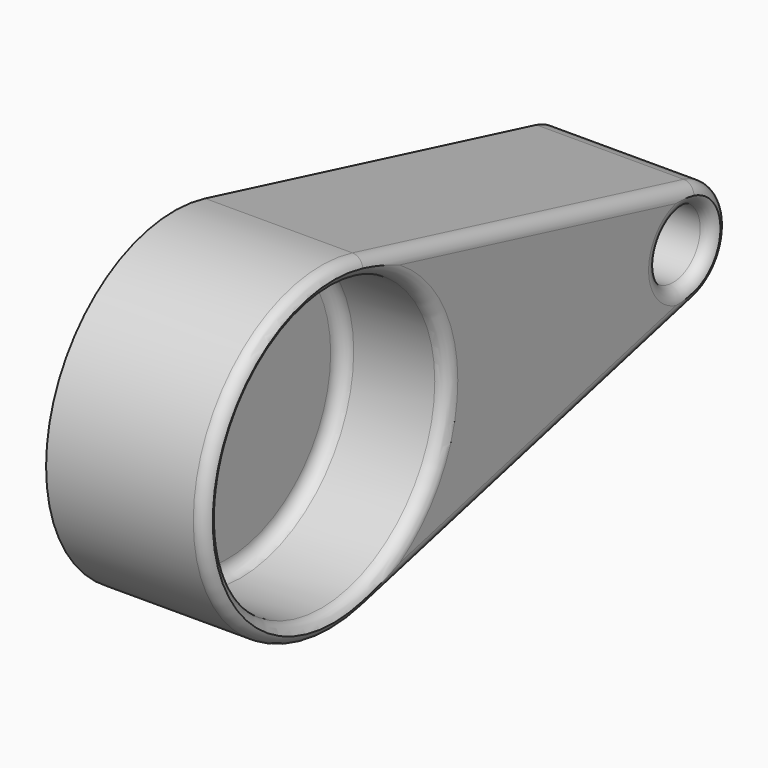
from build123d import *

# Parameters (mm, degrees)
F1_DEPTH     = 75
F2_R         = 66.5
F2_R_2       = 15.875
F3_DEPTH     = 50
F4_T13_ANGLE = 208.0724869359
F4_T16_DEPTH = 200
F4_T19_DEPTH = 200
F4_T22_ANGLE = 151.9275130641
F5_T         = -2.5


# Not quite as in the source:
# - a fillet or chamfer that OpenCascade refuses, or shapes differently, is made with other operations: its cross-section is extruded or revolved along the edge and cut away or added


with BuildPart() as f1:
    # F0 (on Right) → F1 (new body)
    with BuildSketch(Plane.YZ):
        with BuildLine():
            ThreePointArc((18.1901718777, -72.7606875109), (59.1154078512, -46.1559157052), (75, 0))
            ThreePointArc((75, 0), (59.1154078512, 46.1559157052), (18.1901718777, 72.7606875109))
            ThreePointArc((18.1901718777, 72.7606875109), (-75, 0), (18.1901718777, -72.7606875109))
        make_face()
        with BuildLine():
            ThreePointArc((18.1901718777, 72.7606875109), (59.1154078512, 46.1559157052), (75, 0))
            ThreePointArc((75, 0), (59.1154078512, -46.1559157052), (18.1901718777, -72.7606875109))
            Line((18.1901718777, -72.7606875109), (212.2186719068, -24.2535625036))
            ThreePointArc((212.2186719068, -24.2535625036), (181.1552812809, 0), (212.2186719068, 24.2535625036))
            Line((212.2186719068, 24.2535625036), (18.1901718777, 72.7606875109))
        make_face()
        with BuildLine():
            ThreePointArc((231.1552812809, 0), (225.8604172313, 15.3853052351), (212.2186719068, 24.2535625036))
            ThreePointArc((212.2186719068, 24.2535625036), (181.1552812809, 0), (212.2186719068, -24.2535625036))
            ThreePointArc((212.2186719068, -24.2535625036), (225.8604172313, -15.3853052351), (231.1552812809, 0))
        make_face()
    extrude(amount=F1_DEPTH)

    # F2 (on face) → F3 (cut)
    with BuildSketch(Plane.YZ.offset(75)):
        Circle(F2_R)
        with Locations((206.1552812809, 0)):
            Circle(F2_R_2)
    extrude(amount=-F3_DEPTH, mode=Mode.SUBTRACT)

    # F4: fillet of radius 6 on 9 edges, made by hand


with BuildPart() as f4_tool1:
    # F4_s2 → F4_t3 (revolve)
    with BuildSketch(Plane.XY):
        with BuildLine():
            ThreePointArc((31, 66.5), (26.7573593129, 64.7426406871), (25, 60.5))
            Line((25, 60.5), (25, 66.5))
            Line((25, 66.5), (31, 66.5))
        make_face()
    revolve(axis=Axis((25, 0, 0), (1, 0, 0)))


with BuildPart() as f4_tool4:
    # F4_s5 → F4_t6 (revolve)
    with BuildSketch(Plane.XY):
        with BuildLine():
            ThreePointArc((31, 222.0302812809), (26.7573593129, 220.272921968), (25, 216.0302812809))
            Line((25, 216.0302812809), (25, 222.0302812809))
            Line((25, 222.0302812809), (31, 222.0302812809))
        make_face()
    revolve(axis=Axis((25, 206.1552812809, 0), (1, 0, 0)))


with BuildPart() as f1_1:
    add(f1.part)

    # F4_t7: union F4_tool1, F4_tool4
    add([f4_tool1.part, f4_tool4.part])


with BuildPart() as f4_tool8:
    # F4_s9 → F4_t10 (revolve)
    with BuildSketch(Plane.XY):
        with BuildLine():
            ThreePointArc((75, 72.5), (73.2426406871, 68.2573593129), (69, 66.5))
            Line((69, 66.5), (75, 66.5))
            Line((75, 66.5), (75, 72.5))
        make_face()
    revolve(axis=Axis((75, 0, 0), (1, 0, 0)))


with BuildPart() as f4_tool11:
    # F4_s12 → F4_t13 (revolve)
    with BuildSketch(Plane(origin=(0, 0, 0), x_dir=(1, 0, 0), z_dir=(0, 0.9701425001, -0.242535625))):
        with BuildLine():
            ThreePointArc((69, -75), (73.2426406871, -73.2426406871), (75, -69))
            Line((75, -69), (75, -75))
            Line((75, -75), (69, -75))
        make_face()
    revolve(axis=Axis((75, 0, 0), (1, 0, 0)), revolution_arc=F4_T13_ANGLE)


with BuildPart() as f4_tool14:
    # F4_s15 → F4_t16 (new body)
    with BuildSketch(Plane(origin=(0, 194.0285000291, -48.5071250073), x_dir=(1, 0, 0), z_dir=(0, -0.9701425001, 0.242535625))):
        with BuildLine():
            ThreePointArc((69, 75), (73.2426406871, 73.2426406871), (75, 69))
            Line((75, 69), (75, 75))
            Line((75, 75), (69, 75))
        make_face()
    extrude(amount=F4_T16_DEPTH)


with BuildPart() as f4_tool17:
    # F4_s18 → F4_t19 (new body)
    with BuildSketch(Plane(origin=(0, 0, 0), x_dir=(1, 0, 0), z_dir=(0, 0.9701425001, 0.242535625))):
        with BuildLine():
            ThreePointArc((69, 75), (73.2426406871, 73.2426406871), (75, 69))
            Line((75, 69), (75, 75))
            Line((75, 75), (69, 75))
        make_face()
    extrude(amount=F4_T19_DEPTH)


with BuildPart() as f4_tool20:
    # F4_s21 → F4_t22 (revolve)
    with BuildSketch(Plane(origin=(0, 194.0285000291, 48.5071250073), x_dir=(1, 0, 0), z_dir=(0, -0.9701425001, -0.242535625))):
        with BuildLine():
            ThreePointArc((75, -69), (73.2426406871, -73.2426406871), (69, -75))
            Line((69, -75), (75, -75))
            Line((75, -75), (75, -69))
        make_face()
    revolve(axis=Axis((75, 206.1552812809, 0), (1, 0, 0)), revolution_arc=F4_T22_ANGLE)


with BuildPart() as f4_tool23:
    # F4_s24 → F4_t25 (revolve)
    with BuildSketch(Plane.XY):
        with BuildLine():
            ThreePointArc((75, 228.0302812809), (73.2426406871, 223.7876405938), (69, 222.0302812809))
            Line((69, 222.0302812809), (75, 222.0302812809))
            Line((75, 222.0302812809), (75, 228.0302812809))
        make_face()
    revolve(axis=Axis((75, 206.1552812809, 0), (1, 0, 0)))


with BuildPart() as f1_2:
    add(f1_1.part)

    # F4_t26: cut F4_tool8, F4_tool11, F4_tool14, F4_tool17, F4_tool20, F4_tool23
    add([f4_tool8.part, f4_tool11.part, f4_tool14.part, f4_tool17.part, f4_tool20.part, f4_tool23.part], mode=Mode.SUBTRACT)

    # F5
    f5_openings = [f1_2.faces().sort_by_distance(p)[0] for p in [
        (0, 56.613425, 0),
    ]]
    offset(amount=F5_T, openings=f5_openings)


solid = f1_2.part
